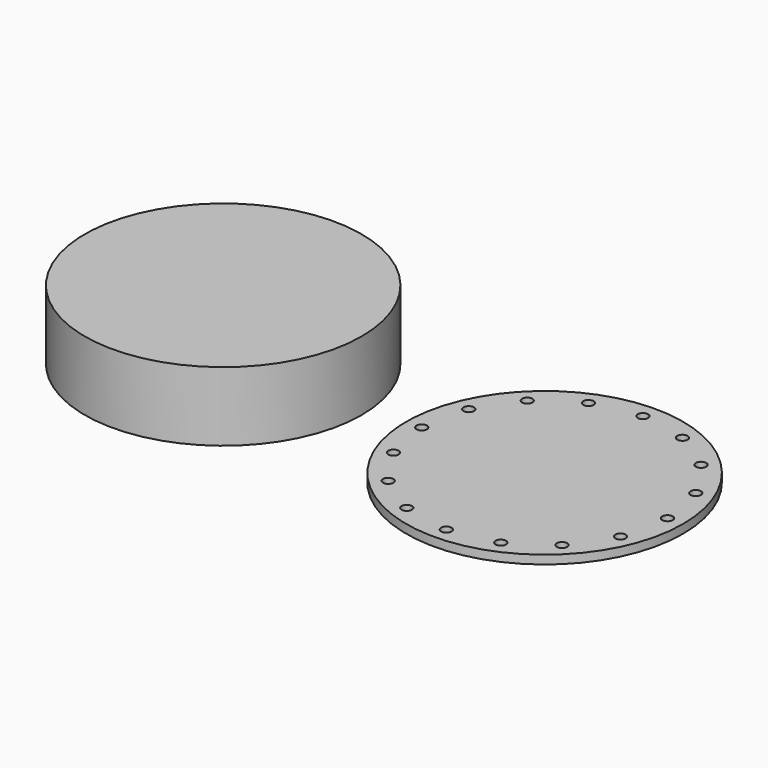
from build123d import *

# Parameters (mm, degrees)
F0_R            = 50.8
F1_DEPTH        = 3.175
F2_R            = 1.905
F3_DEPTH        = 25.4
F3_COPIES_COUNT = 16
F4_R            = 50.8
F5_DEPTH        = 25.4


# Not quite as in the source:
# - a pattern or mirror of a feature is missing from the dataset's text; its kind, count and spacing are read off the source's solid


with BuildPart() as f1:
    # F0 (on Top) → F1 (new body)
    with BuildSketch(Plane.XY):
        Circle(F0_R)
    extrude(amount=F1_DEPTH)

    # F2 (on face) → F3 (cut)
    with BuildSketch(Plane.XY.offset(3.175)):
        with Locations((45.085, 0)):
            Circle(F2_R)
    f3 = extrude(amount=-F3_DEPTH, mode=Mode.SUBTRACT)

    # F3_copies: F3 ×16 about axis
    f3_copies_axis = Axis((0, 0, 0), (0, 0, 1))
    for i in range(1, F3_COPIES_COUNT):
        add(f3.rotate(f3_copies_axis, i * 360 / F3_COPIES_COUNT), mode=Mode.SUBTRACT)


with BuildPart() as f5:
    # F4 (on Top) → F5 (new body)
    with BuildSketch(Plane.XY):
        with Locations((-117.9443001747, 0)):
            Circle(F4_R)
    extrude(amount=F5_DEPTH)


solid = Compound([f1.part, f5.part])
